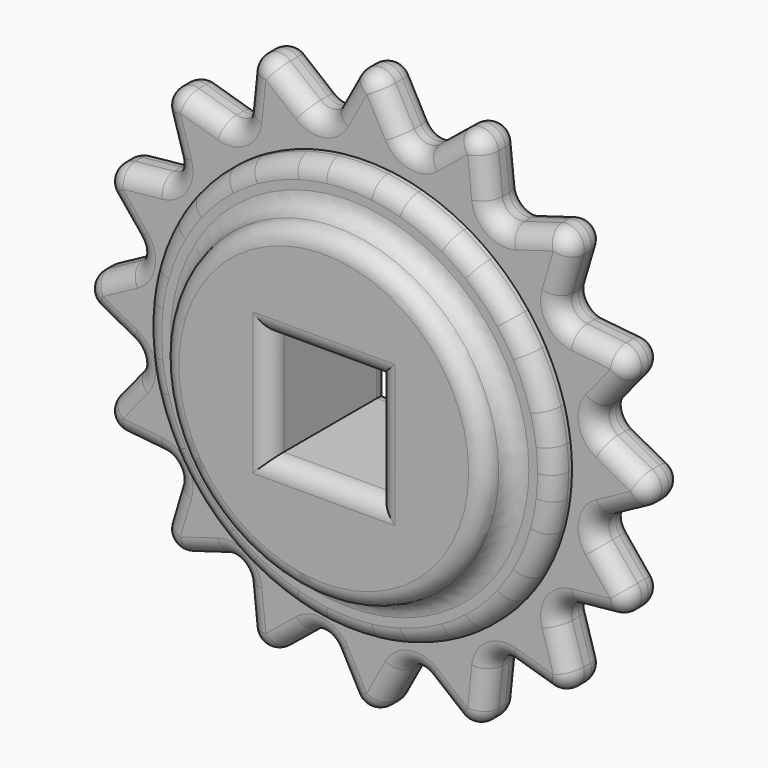
from build123d import *

# Parameters (mm, degrees)
F1_DEPTH = 6.35
F0_R     = 47.8506403027
F2_DEPTH = 12.7
F0_W     = 31.75
F0_H     = 31.75
F3_DEPTH = 22.225
F4_F1_R  = 5.08
F4_F2_R  = 5.08
F5_R     = 5.08
F6_R     = 5.08


with BuildPart() as f1:
    # F0 (on Front) → F1 (new body, symmetric)
    with BuildSketch(Plane.XZ):
        with BuildLine():
            ThreePointArc((-29.6833412919, 52.775745289), (-23.1717268629, 55.9414972561), (-16.3287954603, 58.3073792918))
            Line((-16.3287954603, 58.3073792918), (-12.8704958671, 64.7043521559))
            Line((-12.8704958671, 64.7043521559), (-33.8718805412, 81.7739533857))
            Line((-33.8718805412, 81.7739533857), (-36.6520712769, 54.8537010866))
            Line((-36.6520712769, 54.8537010866), (-29.6833412919, 52.775745289))
        make_face()
        with BuildLine():
            ThreePointArc((-47.620234829, 37.3991079559), (-42.8157683632, 42.8157683632), (-37.3991079559, 47.620234829))
            Line((-37.3991079559, 47.620234829), (-36.6520712769, 54.8537010866))
            Line((-36.6520712769, 54.8537010866), (-62.5870743194, 62.5870743194))
            Line((-62.5870743194, 62.5870743194), (-54.8537010866, 36.6520712769))
            Line((-54.8537010866, 36.6520712769), (-47.620234829, 37.3991079559))
        make_face()
        with BuildLine():
            ThreePointArc((-37.3991079559, 47.620234829), (-33.6401333424, 50.3460174171), (-29.6833412919, 52.775745289))
            Line((-29.6833412919, 52.775745289), (-36.6520712769, 54.8537010866))
            Line((-36.6520712769, 54.8537010866), (-37.3991079559, 47.620234829))
        make_face()
        with BuildLine():
            ThreePointArc((-58.3073792918, 16.3287954603), (-55.9414972561, 23.1717268629), (-52.775745289, 29.6833412919))
            Line((-52.775745289, 29.6833412919), (-54.8537010866, 36.6520712769))
            Line((-54.8537010866, 36.6520712769), (-81.7739533857, 33.8718805412))
            Line((-81.7739533857, 33.8718805412), (-64.7043521559, 12.8704958671))
            Line((-64.7043521559, 12.8704958671), (-58.3073792918, 16.3287954603))
        make_face()
        with BuildLine():
            ThreePointArc((-60.1177538152, -7.2274281233), (-60.5506403027, 0), (-60.1177538152, 7.2274281233))
            Line((-60.1177538152, 7.2274281233), (-64.7043521559, 12.8704958671))
            Line((-64.7043521559, 12.8704958671), (-88.5114893317, 0))
            Line((-88.5114893317, 0), (-64.7043521559, -12.8704958671))
            Line((-64.7043521559, -12.8704958671), (-60.1177538152, -7.2274281233))
        make_face()
        with BuildLine():
            Line((-54.8537010866, -36.6520712769), (-52.775745289, -29.6833412919))
            ThreePointArc((-52.775745289, -29.6833412919), (-55.9414972561, -23.1717268629), (-58.3073792918, -16.3287954603))
            Line((-58.3073792918, -16.3287954603), (-64.7043521559, -12.8704958671))
            Line((-64.7043521559, -12.8704958671), (-81.7739533857, -33.8718805412))
            Line((-81.7739533857, -33.8718805412), (-54.8537010866, -36.6520712769))
        make_face()
        with BuildLine():
            Line((-36.6520712769, -54.8537010866), (-37.3991079559, -47.620234829))
            ThreePointArc((-37.3991079559, -47.620234829), (-42.8157683632, -42.8157683632), (-47.620234829, -37.3991079559))
            Line((-47.620234829, -37.3991079559), (-54.8537010866, -36.6520712769))
            Line((-54.8537010866, -36.6520712769), (-62.5870743194, -62.5870743194))
            Line((-62.5870743194, -62.5870743194), (-36.6520712769, -54.8537010866))
        make_face()
        with BuildLine():
            Line((-12.8704958671, -64.7043521559), (-16.3287954603, -58.3073792918))
            ThreePointArc((-16.3287954603, -58.3073792918), (-23.1717268629, -55.9414972561), (-29.6833412919, -52.775745289))
            Line((-29.6833412919, -52.775745289), (-36.6520712769, -54.8537010866))
            Line((-36.6520712769, -54.8537010866), (-33.8718805412, -81.7739533857))
            Line((-33.8718805412, -81.7739533857), (-12.8704958671, -64.7043521559))
        make_face()
        with BuildLine():
            Line((12.8704958671, -64.7043521559), (7.2274281233, -60.1177538152))
            ThreePointArc((7.2274281233, -60.1177538152), (0, -60.5506403027), (-7.2274281233, -60.1177538152))
            Line((-7.2274281233, -60.1177538152), (-12.8704958671, -64.7043521559))
            Line((-12.8704958671, -64.7043521559), (0, -88.5114893317))
            Line((0, -88.5114893317), (12.8704958671, -64.7043521559))
        make_face()
        with BuildLine():
            Line((36.6520712769, -54.8537010866), (29.6833412919, -52.775745289))
            ThreePointArc((29.6833412919, -52.775745289), (23.1717268629, -55.9414972561), (16.3287954603, -58.3073792918))
            Line((16.3287954603, -58.3073792918), (12.8704958671, -64.7043521559))
            Line((12.8704958671, -64.7043521559), (33.8718805412, -81.7739533857))
            Line((33.8718805412, -81.7739533857), (36.6520712769, -54.8537010866))
        make_face()
        with BuildLine():
            Line((54.8537010866, -36.6520712769), (47.620234829, -37.3991079559))
            ThreePointArc((47.620234829, -37.3991079559), (42.8157683632, -42.8157683632), (37.3991079559, -47.620234829))
            Line((37.3991079559, -47.620234829), (36.6520712769, -54.8537010866))
            Line((36.6520712769, -54.8537010866), (62.5870743194, -62.5870743194))
            Line((62.5870743194, -62.5870743194), (54.8537010866, -36.6520712769))
        make_face()
        with BuildLine():
            Line((64.7043521559, -12.8704958671), (58.3073792918, -16.3287954603))
            ThreePointArc((58.3073792918, -16.3287954603), (55.9414972561, -23.1717268629), (52.775745289, -29.6833412919))
            Line((52.775745289, -29.6833412919), (54.8537010866, -36.6520712769))
            Line((54.8537010866, -36.6520712769), (81.7739533857, -33.8718805412))
            Line((81.7739533857, -33.8718805412), (64.7043521559, -12.8704958671))
        make_face()
        with BuildLine():
            ThreePointArc((60.1177538152, 7.2274281233), (60.4423217958, 3.620190188), (60.5506403027, 0))
            ThreePointArc((60.5506403027, 0), (60.4423217958, -3.620190188), (60.1177538152, -7.2274281233))
            Line((60.1177538152, -7.2274281233), (64.7043521559, -12.8704958671))
            Line((64.7043521559, -12.8704958671), (88.5114893317, 0))
            Line((88.5114893317, 0), (64.7043521559, 12.8704958671))
            Line((64.7043521559, 12.8704958671), (60.1177538152, 7.2274281233))
        make_face()
        with BuildLine():
            ThreePointArc((52.775745289, 29.6833412919), (55.9414972561, 23.1717268629), (58.3073792918, 16.3287954603))
            Line((58.3073792918, 16.3287954603), (64.7043521559, 12.8704958671))
            Line((64.7043521559, 12.8704958671), (81.7739533857, 33.8718805412))
            Line((81.7739533857, 33.8718805412), (54.8537010866, 36.6520712769))
            Line((54.8537010866, 36.6520712769), (52.775745289, 29.6833412919))
        make_face()
        with BuildLine():
            ThreePointArc((37.3991079559, 47.620234829), (42.8157683632, 42.8157683632), (47.620234829, 37.3991079559))
            Line((47.620234829, 37.3991079559), (54.8537010866, 36.6520712769))
            Line((54.8537010866, 36.6520712769), (62.5870743194, 62.5870743194))
            Line((62.5870743194, 62.5870743194), (36.6520712769, 54.8537010866))
            Line((36.6520712769, 54.8537010866), (37.3991079559, 47.620234829))
        make_face()
        with BuildLine():
            ThreePointArc((16.3287954603, 58.3073792918), (23.1717268629, 55.9414972561), (29.6833412919, 52.775745289))
            Line((29.6833412919, 52.775745289), (36.6520712769, 54.8537010866))
            Line((36.6520712769, 54.8537010866), (33.8718805412, 81.7739533857))
            Line((33.8718805412, 81.7739533857), (12.8704958671, 64.7043521559))
            Line((12.8704958671, 64.7043521559), (16.3287954603, 58.3073792918))
        make_face()
        with BuildLine():
            ThreePointArc((-7.2274281233, 60.1177538152), (0, 60.5506403027), (7.2274281233, 60.1177538152))
            Line((7.2274281233, 60.1177538152), (12.8704958671, 64.7043521559))
            Line((12.8704958671, 64.7043521559), (0, 88.5114893317))
            Line((0, 88.5114893317), (-12.8704958671, 64.7043521559))
            Line((-12.8704958671, 64.7043521559), (-7.2274281233, 60.1177538152))
        make_face()
        with BuildLine():
            ThreePointArc((-16.3287954603, 58.3073792918), (-11.8128439149, 59.3871767279), (-7.2274281233, 60.1177538152))
            Line((-7.2274281233, 60.1177538152), (-12.8704958671, 64.7043521559))
            Line((-12.8704958671, 64.7043521559), (-16.3287954603, 58.3073792918))
        make_face()
        with BuildLine():
            ThreePointArc((7.2274281233, 60.1177538152), (11.8128439149, 59.3871767279), (16.3287954603, 58.3073792918))
            Line((16.3287954603, 58.3073792918), (12.8704958671, 64.7043521559))
            Line((12.8704958671, 64.7043521559), (7.2274281233, 60.1177538152))
        make_face()
        with BuildLine():
            ThreePointArc((29.6833412919, 52.775745289), (33.6401333424, 50.3460174171), (37.3991079559, 47.620234829))
            Line((37.3991079559, 47.620234829), (36.6520712769, 54.8537010866))
            Line((36.6520712769, 54.8537010866), (29.6833412919, 52.775745289))
        make_face()
        with BuildLine():
            ThreePointArc((47.620234829, 37.3991079559), (50.3460174171, 33.6401333424), (52.775745289, 29.6833412919))
            Line((52.775745289, 29.6833412919), (54.8537010866, 36.6520712769))
            Line((54.8537010866, 36.6520712769), (47.620234829, 37.3991079559))
        make_face()
        with BuildLine():
            ThreePointArc((58.3073792918, 16.3287954603), (59.3871767279, 11.8128439149), (60.1177538152, 7.2274281233))
            Line((60.1177538152, 7.2274281233), (64.7043521559, 12.8704958671))
            Line((64.7043521559, 12.8704958671), (58.3073792918, 16.3287954603))
        make_face()
        with BuildLine():
            ThreePointArc((-52.775745289, 29.6833412919), (-50.3460174171, 33.6401333424), (-47.620234829, 37.3991079559))
            Line((-47.620234829, 37.3991079559), (-54.8537010866, 36.6520712769))
            Line((-54.8537010866, 36.6520712769), (-52.775745289, 29.6833412919))
        make_face()
        with BuildLine():
            ThreePointArc((-60.1177538152, 7.2274281233), (-59.3871767279, 11.8128439149), (-58.3073792918, 16.3287954603))
            Line((-58.3073792918, 16.3287954603), (-64.7043521559, 12.8704958671))
            Line((-64.7043521559, 12.8704958671), (-60.1177538152, 7.2274281233))
        make_face()
        with BuildLine():
            Line((-64.7043521559, -12.8704958671), (-58.3073792918, -16.3287954603))
            ThreePointArc((-58.3073792918, -16.3287954603), (-59.3871767279, -11.8128439149), (-60.1177538152, -7.2274281233))
            Line((-60.1177538152, -7.2274281233), (-64.7043521559, -12.8704958671))
        make_face()
        with BuildLine():
            Line((-54.8537010866, -36.6520712769), (-47.620234829, -37.3991079559))
            ThreePointArc((-47.620234829, -37.3991079559), (-50.3460174171, -33.6401333424), (-52.775745289, -29.6833412919))
            Line((-52.775745289, -29.6833412919), (-54.8537010866, -36.6520712769))
        make_face()
        with BuildLine():
            Line((-36.6520712769, -54.8537010866), (-29.6833412919, -52.775745289))
            ThreePointArc((-29.6833412919, -52.775745289), (-33.6401333424, -50.3460174171), (-37.3991079559, -47.620234829))
            Line((-37.3991079559, -47.620234829), (-36.6520712769, -54.8537010866))
        make_face()
        with BuildLine():
            Line((-12.8704958671, -64.7043521559), (-7.2274281233, -60.1177538152))
            ThreePointArc((-7.2274281233, -60.1177538152), (-11.8128439149, -59.3871767279), (-16.3287954603, -58.3073792918))
            Line((-16.3287954603, -58.3073792918), (-12.8704958671, -64.7043521559))
        make_face()
        with BuildLine():
            Line((12.8704958671, -64.7043521559), (16.3287954603, -58.3073792918))
            ThreePointArc((16.3287954603, -58.3073792918), (11.8128439149, -59.3871767279), (7.2274281233, -60.1177538152))
            Line((7.2274281233, -60.1177538152), (12.8704958671, -64.7043521559))
        make_face()
        with BuildLine():
            Line((36.6520712769, -54.8537010866), (37.3991079559, -47.620234829))
            ThreePointArc((37.3991079559, -47.620234829), (33.6401333424, -50.3460174171), (29.6833412919, -52.775745289))
            Line((29.6833412919, -52.775745289), (36.6520712769, -54.8537010866))
        make_face()
        with BuildLine():
            Line((54.8537010866, -36.6520712769), (52.775745289, -29.6833412919))
            ThreePointArc((52.775745289, -29.6833412919), (50.3460174171, -33.6401333424), (47.620234829, -37.3991079559))
            Line((47.620234829, -37.3991079559), (54.8537010866, -36.6520712769))
        make_face()
        with BuildLine():
            Line((64.7043521559, -12.8704958671), (60.1177538152, -7.2274281233))
            ThreePointArc((60.1177538152, -7.2274281233), (59.3871767279, -11.8128439149), (58.3073792918, -16.3287954603))
            Line((58.3073792918, -16.3287954603), (64.7043521559, -12.8704958671))
        make_face()
    extrude(amount=F1_DEPTH, both=True)

    # F0 (on Front) → F2 (join, symmetric)
    with BuildSketch(Plane.XZ):
        with BuildLine():
            ThreePointArc((60.1177538152, -7.2274281233), (60.4423217958, -3.620190188), (60.5506403027, 0))
            ThreePointArc((60.5506403027, 0), (60.4423217958, 3.620190188), (60.1177538152, 7.2274281233))
            ThreePointArc((60.1177538152, 7.2274281233), (59.3871767279, 11.8128439149), (58.3073792918, 16.3287954603))
            ThreePointArc((58.3073792918, 16.3287954603), (55.9414972561, 23.1717268629), (52.775745289, 29.6833412919))
            ThreePointArc((52.775745289, 29.6833412919), (50.3460174171, 33.6401333424), (47.620234829, 37.3991079559))
            ThreePointArc((47.620234829, 37.3991079559), (42.8157683632, 42.8157683632), (37.3991079559, 47.620234829))
            ThreePointArc((37.3991079559, 47.620234829), (33.6401333424, 50.3460174171), (29.6833412919, 52.775745289))
            ThreePointArc((29.6833412919, 52.775745289), (23.1717268629, 55.9414972561), (16.3287954603, 58.3073792918))
            ThreePointArc((16.3287954603, 58.3073792918), (11.8128439149, 59.3871767279), (7.2274281233, 60.1177538152))
            ThreePointArc((7.2274281233, 60.1177538152), (0, 60.5506403027), (-7.2274281233, 60.1177538152))
            ThreePointArc((-7.2274281233, 60.1177538152), (-11.8128439149, 59.3871767279), (-16.3287954603, 58.3073792918))
            ThreePointArc((-16.3287954603, 58.3073792918), (-23.1717268629, 55.9414972561), (-29.6833412919, 52.775745289))
            ThreePointArc((-29.6833412919, 52.775745289), (-33.6401333424, 50.3460174171), (-37.3991079559, 47.620234829))
            ThreePointArc((-37.3991079559, 47.620234829), (-42.8157683632, 42.8157683632), (-47.620234829, 37.3991079559))
            ThreePointArc((-47.620234829, 37.3991079559), (-50.3460174171, 33.6401333424), (-52.775745289, 29.6833412919))
            ThreePointArc((-52.775745289, 29.6833412919), (-55.9414972561, 23.1717268629), (-58.3073792918, 16.3287954603))
            ThreePointArc((-58.3073792918, 16.3287954603), (-59.3871767279, 11.8128439149), (-60.1177538152, 7.2274281233))
            ThreePointArc((-60.1177538152, 7.2274281233), (-60.5506403027, 0), (-60.1177538152, -7.2274281233))
            ThreePointArc((-60.1177538152, -7.2274281233), (-59.3871767279, -11.8128439149), (-58.3073792918, -16.3287954603))
            ThreePointArc((-58.3073792918, -16.3287954603), (-55.9414972561, -23.1717268629), (-52.775745289, -29.6833412919))
            ThreePointArc((-52.775745289, -29.6833412919), (-50.3460174171, -33.6401333424), (-47.620234829, -37.3991079559))
            ThreePointArc((-47.620234829, -37.3991079559), (-42.8157683632, -42.8157683632), (-37.3991079559, -47.620234829))
            ThreePointArc((-37.3991079559, -47.620234829), (-33.6401333424, -50.3460174171), (-29.6833412919, -52.775745289))
            ThreePointArc((-29.6833412919, -52.775745289), (-23.1717268629, -55.9414972561), (-16.3287954603, -58.3073792918))
            ThreePointArc((-16.3287954603, -58.3073792918), (-11.8128439149, -59.3871767279), (-7.2274281233, -60.1177538152))
            ThreePointArc((-7.2274281233, -60.1177538152), (0, -60.5506403027), (7.2274281233, -60.1177538152))
            ThreePointArc((7.2274281233, -60.1177538152), (11.8128439149, -59.3871767279), (16.3287954603, -58.3073792918))
            ThreePointArc((16.3287954603, -58.3073792918), (23.1717268629, -55.9414972561), (29.6833412919, -52.775745289))
            ThreePointArc((29.6833412919, -52.775745289), (33.6401333424, -50.3460174171), (37.3991079559, -47.620234829))
            ThreePointArc((37.3991079559, -47.620234829), (42.8157683632, -42.8157683632), (47.620234829, -37.3991079559))
            ThreePointArc((47.620234829, -37.3991079559), (50.3460174171, -33.6401333424), (52.775745289, -29.6833412919))
            ThreePointArc((52.775745289, -29.6833412919), (55.9414972561, -23.1717268629), (58.3073792918, -16.3287954603))
            ThreePointArc((58.3073792918, -16.3287954603), (59.3871767279, -11.8128439149), (60.1177538152, -7.2274281233))
        make_face()
        Circle(F0_R, mode=Mode.SUBTRACT)
    extrude(amount=F2_DEPTH, both=True)

    # F0 (on Front) → F3 (join, symmetric)
    with BuildSketch(Plane.XZ):
        Circle(F0_R)
        Rectangle(F0_W, F0_H, mode=Mode.SUBTRACT)
    extrude(amount=F3_DEPTH, both=True)

    # F4: fillet of radius 5.08 on 64 edges, made by hand

    # F4_f1
    f4_f1_edges = [f1.edges().sort_by_distance(p)[0] for p in [
        (-54.8537010866, 0, 36.6520712769),
        (-36.6520712769, 0, 54.8537010866),
        (-12.8704958671, 0, 64.7043521559),
        (12.8704958671, 0, 64.7043521559),
        (36.6520712769, 0, 54.8537010866),
        (54.8537010866, 0, 36.6520712769),
        (64.7043521559, 0, 12.8704958671),
        (64.7043521559, 0, -12.8704958671),
        (54.8537010866, 0, -36.6520712769),
        (36.6520712769, 0, -54.8537010866),
        (12.8704958671, 0, -64.7043521559),
        (-12.8704958671, 0, -64.7043521559),
        (-36.6520712769, 0, -54.8537010866),
        (-54.8537010866, 0, -36.6520712769),
        (-64.7043521559, 0, -12.8704958671),
        (-64.7043521559, 0, 12.8704958671),
    ]]
    fillet(f4_f1_edges, radius=F4_F1_R)

    # F4_f2
    f4_f2_edges = [f1.edges().sort_by_distance(p)[0] for p in [
        (-71.3628935622, 6.35, 34.947083394),
        (-81.7739533857, 0, 33.8718805412),
        (-71.3628935622, -6.35, 34.947083394),
        (-52.5570469185, 6.35, 59.5962921206),
        (-62.5870743194, 0, 62.5870743194),
        (-52.5570469185, -6.35, 59.5962921206),
        (-25.7498663123, 6.35, 75.1725056135),
        (-33.8718805412, 0, 81.7739533857),
        (-25.7498663123, -6.35, 75.1725056135),
        (4.9774980168, 6.35, 79.3043865673),
        (0, 0, 88.5114893317),
        (4.9774980168, -6.35, 79.3043865673),
        (34.947083394, 6.35, 71.3628935622),
        (33.8718805412, 0, 81.7739533857),
        (34.947083394, -6.35, 71.3628935622),
        (59.5962921206, 6.35, 52.5570469185),
        (62.5870743194, 0, 62.5870743194),
        (59.5962921206, -6.35, 52.5570469185),
        (75.1725056135, 6.35, 25.7498663123),
        (81.7739533857, 0, 33.8718805412),
        (75.1725056135, -6.35, 25.7498663123),
        (79.3043865673, 6.35, -4.9774980168),
        (88.5114893317, 0, 0),
        (79.3043865673, -6.35, -4.9774980168),
        (71.3628935622, 6.35, -34.947083394),
        (81.7739533857, 0, -33.8718805412),
        (71.3628935622, -6.35, -34.947083394),
        (52.5570469185, 6.35, -59.5962921206),
        (62.5870743194, 0, -62.5870743194),
        (52.5570469185, -6.35, -59.5962921206),
        (25.7498663123, 6.35, -75.1725056135),
        (33.8718805412, 0, -81.7739533857),
        (25.7498663123, -6.35, -75.1725056135),
        (-4.9774980168, 6.35, -79.3043865673),
        (0, 0, -88.5114893317),
        (-4.9774980168, -6.35, -79.3043865673),
        (-34.947083394, 6.35, -71.3628935622),
        (-33.8718805412, 0, -81.7739533857),
        (-34.947083394, -6.35, -71.3628935622),
        (-59.5962921206, 6.35, -52.5570469185),
        (-62.5870743194, 0, -62.5870743194),
        (-59.5962921206, -6.35, -52.5570469185),
        (-75.1725056135, 6.35, -25.7498663123),
        (-81.7739533857, 0, -33.8718805412),
        (-75.1725056135, -6.35, -25.7498663123),
        (-79.3043865673, 6.35, 4.9774980168),
        (-88.5114893317, 0, 0),
        (-79.3043865673, -6.35, 4.9774980168),
        (-67.5307786711, -6.35, 13.4327070565),
        (-67.5307786711, 6.35, 13.4327070565),
        (-67.5307786711, -6.35, -13.4327070565),
        (-67.5307786711, 6.35, -13.4327070565),
        (-57.2498297865, -6.35, -38.2531132878),
        (-57.2498297865, 6.35, -38.2531132878),
        (-38.2531132878, -6.35, -57.2498297865),
        (-38.2531132878, 6.35, -57.2498297865),
        (-13.4327070565, -6.35, -67.5307786711),
        (-13.4327070565, 6.35, -67.5307786711),
        (13.4327070565, -6.35, -67.5307786711),
        (13.4327070565, 6.35, -67.5307786711),
        (38.2531132878, -6.35, -57.2498297865),
        (38.2531132878, 6.35, -57.2498297865),
        (57.2498297865, -6.35, -38.2531132878),
        (57.2498297865, 6.35, -38.2531132878),
        (67.5307786711, -6.35, -13.4327070565),
        (67.5307786711, 6.35, -13.4327070565),
        (67.5307786711, -6.35, 13.4327070565),
        (67.5307786711, 6.35, 13.4327070565),
        (57.2498297865, -6.35, 38.2531132878),
        (57.2498297865, 6.35, 38.2531132878),
        (38.2531132878, -6.35, 57.2498297865),
        (38.2531132878, 6.35, 57.2498297865),
        (13.4327070565, -6.35, 67.5307786711),
        (13.4327070565, 6.35, 67.5307786711),
        (-13.4327070565, -6.35, 67.5307786711),
        (-13.4327070565, 6.35, 67.5307786711),
        (-38.2531132878, -6.35, 57.2498297865),
        (-38.2531132878, 6.35, 57.2498297865),
        (-57.2498297865, -6.35, 38.2531132878),
        (-57.2498297865, 6.35, 38.2531132878),
    ]]
    fillet(f4_f2_edges, radius=F4_F2_R)

    # F5
    f5_edges = [f1.edges().sort_by_distance(p)[0] for p in [
        (-47.85064, -22.225, 0),
        (-15.875, -22.225, 0),
        (0, -22.225, 15.875),
        (15.875, -22.225, 0),
        (0, -22.225, -15.875),
        (-47.85064, 22.225, 0),
        (-15.875, 22.225, 0),
        (0, 22.225, 15.875),
        (15.875, 22.225, 0),
        (0, 22.225, -15.875),
    ]]
    fillet(f5_edges, radius=F5_R)

    # F6
    f6_edges = [f1.edges().sort_by_distance(p)[0] for p in [
        (-16.328795, -12.7, 58.307379),
        (-47.85064, -12.7, 0),
        (-16.328795, 12.7, 58.307379),
        (-47.85064, 12.7, 0),
    ]]
    fillet(f6_edges, radius=F6_R)


solid = f1.part
